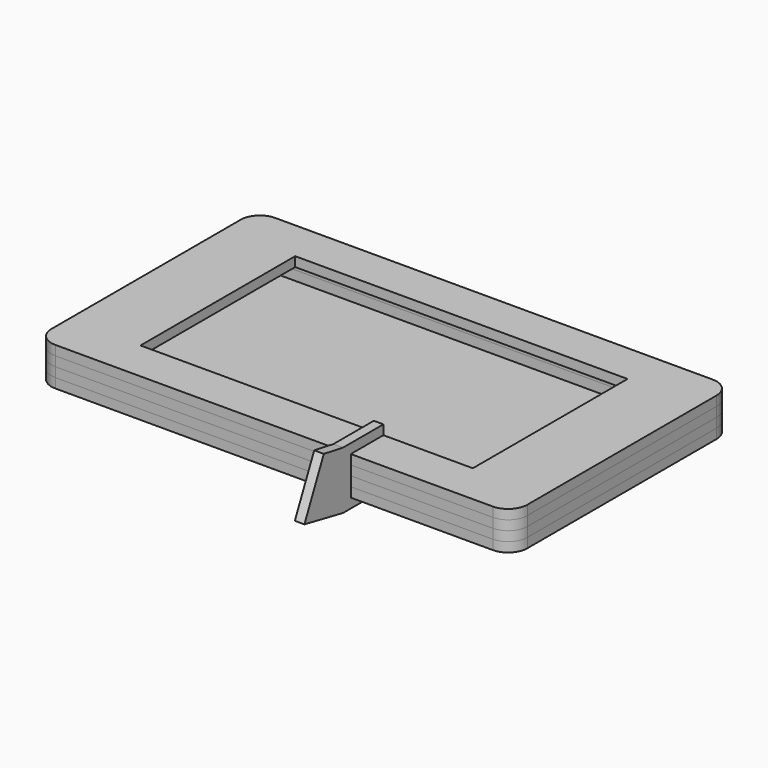
from build123d import *

# Parameters (mm, degrees)
F0_W      = 110
F0_H      = 64
F1_DEPTH  = 3.175
F2_W      = 137.5
F2_H      = 71
F3_DEPTH  = 3.175
F4_W      = 137.5
F4_H      = 71
F5_DEPTH  = 3.175
F6_W      = 110
F6_H      = 64
F7_DEPTH  = 3.175
F13_DEPTH = 3.175


# Not quite as in the source:
# - a length typed as a fraction of an inch, garbled in the dataset ("3 / 203.2 mm" for 3/8 in), is restored


with BuildPart() as f1:
    # F0 (on Top) → F1 (new body)
    with BuildSketch(Plane.XY):
        with BuildLine():
            Line((0, 35.5), (68.75, 35.5))
            Line((68.75, 35.5), (68.75, 0))
            Line((68.75, 0), (78.75, 0))
            Line((78.75, 0), (78.75, 39.15))
            ThreePointArc((78.75, 39.15), (76.8901280605, 43.6401280605), (72.4, 45.5))
            Line((72.4, 45.5), (0, 45.5))
            Line((0, 45.5), (0, 35.5))
        make_face()
        with BuildLine():
            Line((-68.75, 35.5), (0, 35.5))
            Line((0, 35.5), (0, 45.5))
            Line((0, 45.5), (-72.4, 45.5))
            ThreePointArc((-72.4, 45.5), (-76.8901280605, 43.6401280605), (-78.75, 39.15))
            Line((-78.75, 39.15), (-78.75, 0))
            Line((-78.75, 0), (-68.75, 0))
            Line((-68.75, 0), (-68.75, 35.5))
        make_face()
        with BuildLine():
            Line((78.75, 0), (68.75, 0))
            Line((68.75, 0), (68.75, -35.5))
            Line((68.75, -35.5), (0, -35.5))
            Line((0, -35.5), (0, -45.5))
            Line((0, -45.5), (72.4, -45.5))
            ThreePointArc((72.4, -45.5), (76.8901280605, -43.6401280605), (78.75, -39.15))
            Line((78.75, -39.15), (78.75, 0))
        make_face()
        with BuildLine():
            Line((-68.75, -35.5), (-68.75, 0))
            Line((-68.75, 0), (-78.75, 0))
            Line((-78.75, 0), (-78.75, -39.15))
            ThreePointArc((-78.75, -39.15), (-76.8901280605, -43.6401280605), (-72.4, -45.5))
            Line((-72.4, -45.5), (0, -45.5))
            Line((0, -45.5), (0, -35.5))
            Line((0, -35.5), (-68.75, -35.5))
        make_face()
        Polygon((68.75, 0), (68.75, 35.5), (0, 35.5), (-68.75, 35.5), (-68.75, 0), (-68.75, -35.5), (0, -35.5), (68.75, -35.5), align=None)
        Rectangle(F0_W, F0_H, mode=Mode.SUBTRACT)
        Rectangle(F0_W, F0_H)
    extrude(amount=F1_DEPTH)


with BuildPart() as f3:
    # F2 (on face) → F3 (new body)
    with BuildSketch(Plane.XY.offset(3.175)):
        with BuildLine():
            Line((-72.4, -45.5), (72.4, -45.5))
            ThreePointArc((72.4, -45.5), (76.8901280605, -43.6401280605), (78.75, -39.15))
            Line((78.75, -39.15), (78.75, 39.15))
            ThreePointArc((78.75, 39.15), (76.8901280605, 43.6401280605), (72.4, 45.5))
            Line((72.4, 45.5), (-72.4, 45.5))
            ThreePointArc((-72.4, 45.5), (-76.8901280605, 43.6401280605), (-78.75, 39.15))
            Line((-78.75, 39.15), (-78.75, -39.15))
            ThreePointArc((-78.75, -39.15), (-76.8901280605, -43.6401280605), (-72.4, -45.5))
        make_face()
        Rectangle(F2_W, F2_H, mode=Mode.SUBTRACT)
    extrude(amount=F3_DEPTH)


with BuildPart() as f5:
    # F4 (on face) → F5 (new body)
    with BuildSketch(Plane.XY.offset(6.35)):
        with BuildLine():
            ThreePointArc((-78.75, -39.15), (-76.8901280605, -43.6401280605), (-72.4, -45.5))
            Line((-72.4, -45.5), (72.4, -45.5))
            ThreePointArc((72.4, -45.5), (76.8901280605, -43.6401280605), (78.75, -39.15))
            Line((78.75, -39.15), (78.75, 39.15))
            ThreePointArc((78.75, 39.15), (76.8901280605, 43.6401280605), (72.4, 45.5))
            Line((72.4, 45.5), (-72.4, 45.5))
            ThreePointArc((-72.4, 45.5), (-76.8901280605, 43.6401280605), (-78.75, 39.15))
            Line((-78.75, 39.15), (-78.75, -39.15))
        make_face()
        Rectangle(F4_W, F4_H, mode=Mode.SUBTRACT)
    extrude(amount=F5_DEPTH)


with BuildPart() as f7:
    # F6 (on face) → F7 (new body)
    with BuildSketch(Plane.XY.offset(9.525)):
        with BuildLine():
            Line((-72.4, -45.5), (72.4, -45.5))
            ThreePointArc((72.4, -45.5), (76.8901280605, -43.6401280605), (78.75, -39.15))
            Line((78.75, -39.15), (78.75, 39.15))
            ThreePointArc((78.75, 39.15), (76.8901280605, 43.6401280605), (72.4, 45.5))
            Line((72.4, 45.5), (-72.4, 45.5))
            ThreePointArc((-72.4, 45.5), (-76.8901280605, 43.6401280605), (-78.75, 39.15))
            Line((-78.75, 39.15), (-78.75, -39.15))
            ThreePointArc((-78.75, -39.15), (-76.8901280605, -43.6401280605), (-72.4, -45.5))
        make_face()
        Rectangle(F6_W, F6_H, mode=Mode.SUBTRACT)
    extrude(amount=F7_DEPTH)


with BuildPart() as f13:
    # F12 (on line) → F13 (new body)
    with BuildSketch(Plane(origin=(25.4, 0, 0), x_dir=(0, -1, 0), z_dir=(-1, 0, 0))):
        Polygon((56.6581731759, 17.2826488226), (48.675, 15.875), (48.675, -3.175), (64.6714465192, 0), align=None)
        Polygon((48.675, -3.175), (48.675, 15.875), (32, 15.875), (32, 12.7), (45.5, 12.7), (45.5, 0), (32, 0), (32, -3.175), align=None)
    extrude(amount=F13_DEPTH)


solid = Compound([f1.part, f3.part, f5.part, f7.part, f13.part])
